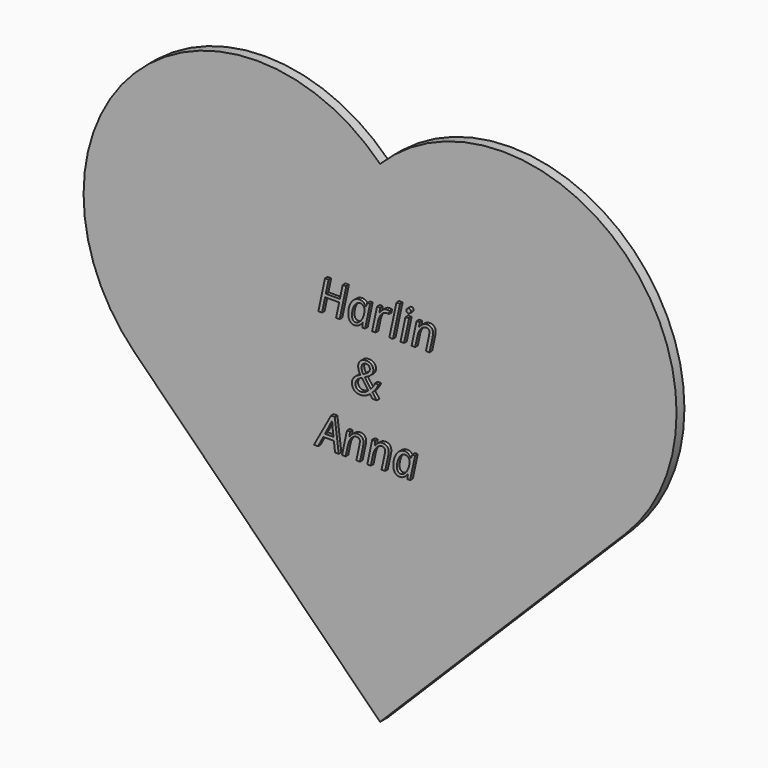
from build123d import *

# Parameters (mm, degrees)
F1_DEPTH     = 1.524
F2_TEXT_SIZE = 6.7773275077
F3_DEPTH     = 0.508


# Not quite as in the source:
# - Text() gives the source's letters only with a copy of the font that has no kerning and outlines rounded to 1/6400 em; it was checked with that copy


with BuildPart() as f1:
    # F0 (on Front) → F1 (new body)
    with BuildSketch(Plane.XZ):
        with BuildLine():
            Line((-38.1, 38.1000037242), (0, 0))
            Line((0, 0), (38.1, 38.1000037242))
            ThreePointArc((38.1, 38.1000037242), (38.0999981379, 76.2000018621), (0, 76.2))
            ThreePointArc((0, 76.2), (-38.0999981379, 76.2000018621), (-38.1, 38.1000037242))
        make_face()
    extrude(amount=F1_DEPTH)

    # F2 (on face) → F3 (join)
    with BuildSketch(Plane.XZ.offset(1.524)):
        with Locations((-9.451195001, 53.289167583)):
            Text('Harlin', F2_TEXT_SIZE, font='Open Sans', font_style=FontStyle.ITALIC, text_align=(TextAlign.LEFT, TextAlign.BOTTOM))
        with Locations((-4.1680564173, 44.0720021725)):
            Text('&', F2_TEXT_SIZE, font='Open Sans', font_style=FontStyle.ITALIC, text_align=(TextAlign.LEFT, TextAlign.BOTTOM))
        with Locations((-9.451195001, 34.854836762)):
            Text('Anna', F2_TEXT_SIZE, font='Open Sans', font_style=FontStyle.ITALIC, text_align=(TextAlign.LEFT, TextAlign.BOTTOM))
    extrude(amount=F3_DEPTH)


solid = f1.part
